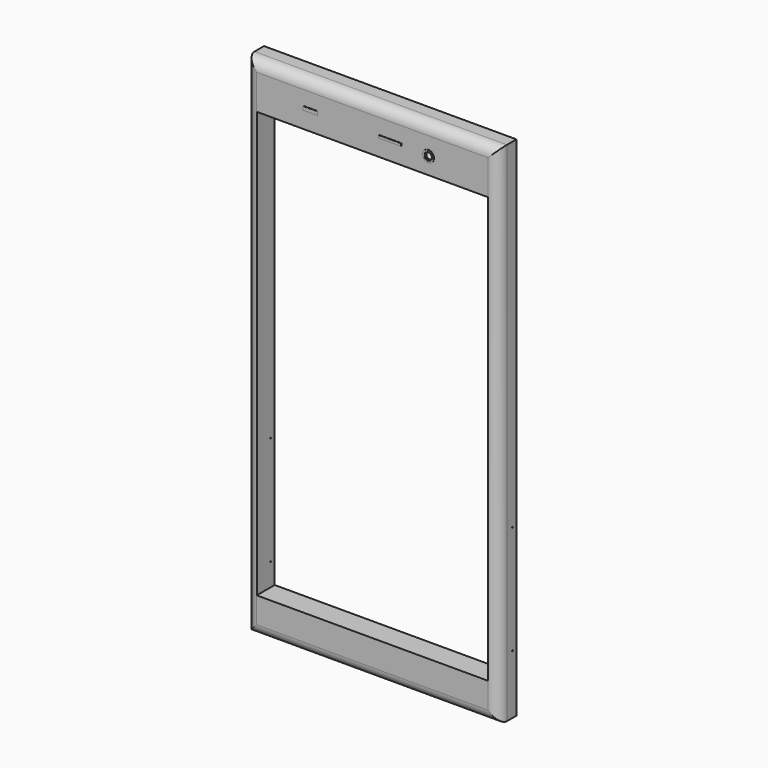
from build123d import *

# Parameters (mm, degrees)
F0_W      = 72.1
F0_H      = 144.9
F0_W_2    = 65.9861192107
F0_H_2    = 121.5704865754
F1_DEPTH  = 6.4
F2_R      = 3
F3_R      = 1.6199699766
F3_R_2    = 1.0969181454
F3_W      = 6.3781980425
F3_H      = 0.7731094956
F3_W_2    = 4.1554919444
F3_H_2    = 1.0630339384
F4_DEPTH  = 0.1
F6_D      = 0.28
F13_D     = 2
F13_DEPTH = 0.5
F13_TIP   = 0.600860619


# Not quite as in the source:
# - the program builds the solid bodies; features that only make, move or delete a surface that nothing else refers to are left out


with BuildPart() as f1:
    # F0 (on Front) → F1 (new body)
    with BuildSketch(Plane.XZ):
        with Locations((21.9475186944, 24.6742434323)):
            Rectangle(F0_W, F0_H)
        with Locations((21.9411961734, 23.4142001718)):
            Rectangle(F0_W_2, F0_H_2, mode=Mode.SUBTRACT)
    extrude(amount=F1_DEPTH)

    # F2
    f2_edges = [f1.edges().sort_by_distance(p)[0] for p in [
        (21.947519, -6.4, 97.124243),
        (-14.102481, -6.4, 24.674243),
        (21.947519, -6.4, -47.775757),
        (57.997519, -6.4, 24.674243),
    ]]
    fillet(f2_edges, radius=F2_R)

    # F3 (on face) → F4 (join, symmetric)
    with BuildSketch(Plane.XZ.offset(6.4)):
        with Locations((37.9579253495, 88.9658480883)):
            Circle(F3_R)
        with Locations((37.9579253495, 88.9658480883)):
            Circle(F3_R_2, mode=Mode.SUBTRACT)
        with Locations((27.0376754925, 89.3524028361)):
            Rectangle(F3_W, F3_H)
        with Locations((4.2791056912, 89.4973650575)):
            Rectangle(F3_W_2, F3_H_2)
    extrude(amount=F4_DEPTH, both=True)

    # F6 (through all)
    with Locations(Plane.YZ.offset(57.9975186944)):
        with Locations((-1.4492898481, -30.8446902782), (-1.4492898481, 0.1785024215)):
            Hole(F6_D / 2)

    # F13
    with Locations(Plane.XZ.offset(6.4)):
        with Locations((37.9579253495, 88.9658480883)):
            Hole(F13_D / 2, depth=F13_DEPTH)
            with Locations((0, 0, -(F13_DEPTH + F13_TIP / 2))):  # 118° drill point
                Cone(0, F13_D / 2, F13_TIP, mode=Mode.SUBTRACT)


solid = f1.part
